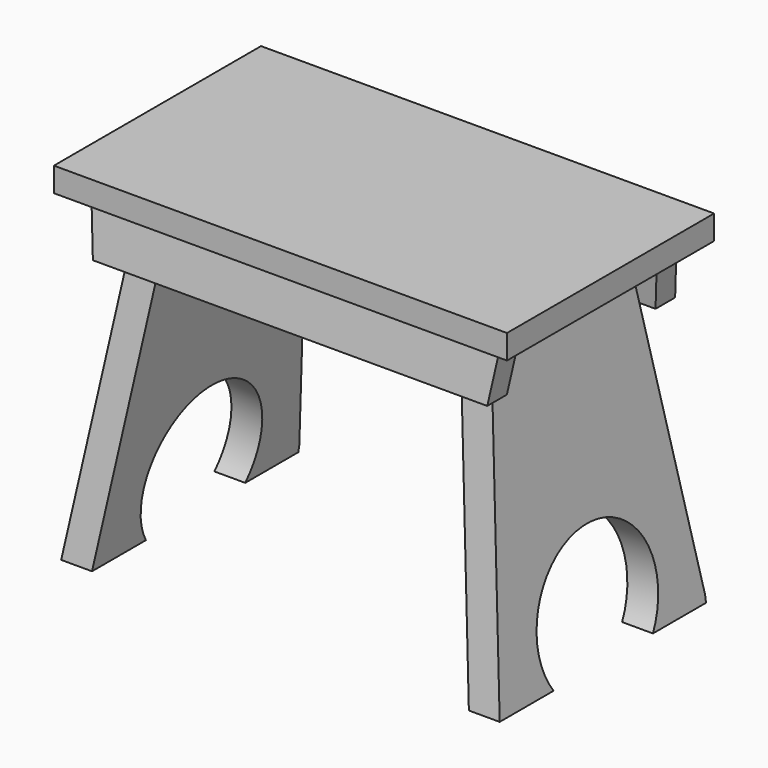
from build123d import *

# Parameters (mm, degrees)
F1_DEPTH       = 101.6
F2_DEPTH       = 101.6
F2_DEPTH_BACK  = 100.838
F4_DEPTH       = 177.801
F4_DEPTH_BACK  = 177.801
F6_DEPTH       = 101.601
F6_DEPTH_BACK  = 101.601
F7_DEPTH       = 101.601
F7_DEPTH_BACK  = 101.601
F8_DEPTH       = 161.798
F8_DEPTH_BACK  = 161.798
F9_DEPTH       = 161.798
F9_DEPTH_BACK  = 161.798
F10_DEPTH      = 101.601
F10_DEPTH_BACK = 101.601


# Not quite as in the source:
# - a feature names something its author has since deleted; it is built from what else it names


with BuildPart() as f1:
    # F0 (on Front) → F1 (new body, symmetric)
    with BuildSketch(Plane.XZ):
        Polygon((177.8, -9.525), (177.8, 9.525), (-177.8, 9.525), (-177.8, -9.525), (-160.77771832, -9.525), (-136.7410615279, -9.525), (-112.5340089202, -9.525), (112.5340089202, -9.525), (136.7410615279, -9.525), (160.77771832, -9.525), align=None)
    extrude(amount=F1_DEPTH, both=True)

    # F0 (on Front) → F6 (cut, two sides)
    with BuildSketch(Plane.XZ) as f6_sk:
        Polygon((177.8, -52.5049223718), (177.8, -9.525), (160.77771832, -9.525), (154.7372841544, -52.5049223718), align=None)
    extrude(amount=F6_DEPTH, mode=Mode.SUBTRACT)
    extrude(f6_sk.sketch, amount=-F6_DEPTH_BACK, mode=Mode.SUBTRACT)

    # F0 (on Front) → F7 (cut, two sides)
    with BuildSketch(Plane.XZ) as f7_sk:
        Polygon((-160.77771832, -9.525), (-177.8, -9.525), (-177.8, -52.5049223718), (-154.7372841544, -52.5049223718), align=None)
    extrude(amount=F7_DEPTH, mode=Mode.SUBTRACT)
    extrude(f7_sk.sketch, amount=-F7_DEPTH_BACK, mode=Mode.SUBTRACT)


with BuildPart() as f2:
    # F0 (on Front) → F2 (new body, two sides)
    with BuildSketch(Plane.XZ) as f2_sk:
        Polygon((-118.5744430858, -52.5049223718), (-142.7814956935, -52.5049223718), (-172.0910291718, -261.0530894604), (-147.883976564, -261.0530894604), align=None)
        Polygon((-112.5340089202, -9.525), (-136.7410615279, -9.525), (-142.7814956935, -52.5049223718), (-118.5744430858, -52.5049223718), align=None)
    extrude(amount=F2_DEPTH)
    extrude(f2_sk.sketch, amount=-F2_DEPTH_BACK)


with BuildPart() as f2b:
    # F0 (on Front) → F2, piece 2 (new body, two sides)
    with BuildSketch(Plane.XZ) as f2_2_sk:
        Polygon((142.7814956935, -52.5049223718), (136.7410615279, -9.525), (112.5340089202, -9.525), (118.5744430858, -52.5049223718), align=None)
        Polygon((172.0910291718, -261.0530894604), (142.7814956935, -52.5049223718), (118.5744430858, -52.5049223718), (147.883976564, -261.0530894604), align=None)
    extrude(amount=F2_DEPTH)
    extrude(f2_2_sk.sketch, amount=-F2_DEPTH_BACK)


with BuildPart() as f4_tool:
    # F3 (on Right) → F4 (new body, two sides)
    with BuildSketch(Plane.YZ) as f4_sk:
        Polygon((100.838, -255.6311777319), (100.838, -9.525), (66.2500323562, -9.525), align=None)
        Polygon((-101.6, -261.0530894604), (-66.2500323562, -9.525), (-101.6, -9.525), align=None)
        with BuildLine():
            Line((-48.7405628211, -261.0530894604), (48.7405628211, -261.0530894604))
            ThreePointArc((48.7405628211, -261.0530894604), (0, -169.4420519551), (-48.7405628211, -261.0530894604))
        make_face()
    extrude(amount=F4_DEPTH)
    extrude(f4_sk.sketch, amount=-F4_DEPTH_BACK)


with BuildPart() as f2_1:
    add(f2.part)

    # F4: cut by f4_tool
    add(f4_tool.part, mode=Mode.SUBTRACT)


with BuildPart() as f2b_1:
    add(f2b.part)

    # F4: cut by f4_tool
    add(f4_tool.part, mode=Mode.SUBTRACT)


with BuildPart() as f8:
    # F5 (on Right) → F8 (new body, two sides)
    with BuildSketch(Plane.YZ) as f8_sk:
        Polygon((-72.9137584568, -52.213318646), (-66.9143065223, -9.525), (-86.1515217788, -9.525), (-92.1509737133, -52.213318646), align=None)
    extrude(amount=F8_DEPTH)
    extrude(f8_sk.sketch, amount=-F8_DEPTH_BACK)


with BuildPart() as f9:
    # F5 (on Right) → F9 (new body, two sides)
    with BuildSketch(Plane.YZ) as f9_sk:
        Polygon((66.9143065223, -9.525), (72.9137584568, -52.213318646), (92.1509737133, -52.213318646), (86.1515217788, -9.525), align=None)
    extrude(amount=F9_DEPTH)
    extrude(f9_sk.sketch, amount=-F9_DEPTH_BACK)


with BuildPart() as f10_tool:
    # F0 (on Front) → F10 (new body, two sides)
    with BuildSketch(Plane.XZ) as f10_sk:
        Polygon((177.8, -52.5049223718), (177.8, -9.525), (160.77771832, -9.525), (154.7372841544, -52.5049223718), align=None)
        Polygon((-160.77771832, -9.525), (-177.8, -9.525), (-177.8, -52.5049223718), (-154.7372841544, -52.5049223718), align=None)
    extrude(amount=F10_DEPTH)
    extrude(f10_sk.sketch, amount=-F10_DEPTH_BACK)


with BuildPart() as f8_1:
    add(f8.part)

    # F10: cut by f10_tool
    add(f10_tool.part, mode=Mode.SUBTRACT)

    # F11: cut F2, F2b
    add(f2_1.part, mode=Mode.SUBTRACT)
    add(f2b_1.part, mode=Mode.SUBTRACT)


with BuildPart() as f9_1:
    add(f9.part)

    # F10: cut by f10_tool
    add(f10_tool.part, mode=Mode.SUBTRACT)

    # F11: cut F2, F2b
    add(f2_1.part, mode=Mode.SUBTRACT)
    add(f2b_1.part, mode=Mode.SUBTRACT)


solid = Compound([f1.part, f2_1.part, f2b_1.part, f8_1.part, f9_1.part])
